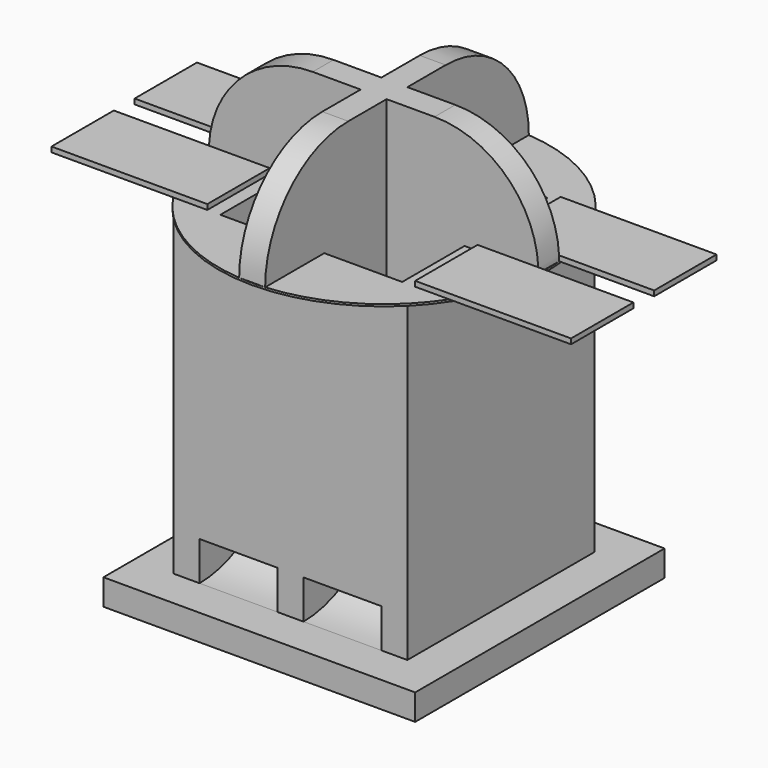
from build123d import *

# Parameters (mm, degrees)
F0_W          = 76.2
F0_H          = 76.2
F1_DEPTH      = 6.35
F2_W          = 57.15
F2_H          = 57.15
F3_DEPTH      = 76.2
F4_W          = 19.05
F4_H          = 19.05
F5_DEPTH      = 76.2
F5_DEPTH_BACK = 25.4
F7_W          = 19.05
F7_H          = 9.525
F6_W          = 19.05
F6_H          = 9.525
F8_DEPTH      = 6.35
F9_DEPTH      = 6.35
F10_R         = 25.4
F12_DEPTH     = 0.508
F13_DEPTH     = 25.4
F15_DEPTH     = 1.27
F16_W         = 6.35
F16_H         = 6.35
F17_DEPTH     = 25.4
F18_T1_DEPTH  = 6.35
F18_T3_DEPTH  = 6.35


# Not quite as in the source:
# - a fillet or chamfer that OpenCascade refuses, or shapes differently, is made with other operations: its cross-section is extruded or revolved along the edge and cut away or added


with BuildPart() as f1:
    # F0 (on Top) → F1 (new body)
    with BuildSketch(Plane.XY):
        with Locations((-41.2033051252, 20.37120983)):
            Rectangle(F0_W, F0_H)
    extrude(amount=F1_DEPTH)

    # F2 (on face) → F3 (join)
    with BuildSketch(Plane.XY.offset(6.35)):
        with Locations((-41.2033051252, 20.37120983)):
            Rectangle(F2_W, F2_H)
    extrude(amount=F3_DEPTH)

    # F4 (on face) → F5 (cut, two sides)
    with BuildSketch(Plane.XY.offset(82.55)) as f5_sk:
        with Locations((-53.9033051252, 33.07120983)):
            Rectangle(F4_W, F4_H)
        with Locations((-28.5033051252, 33.07120983)):
            Rectangle(F4_W, F4_H)
        with Locations((-28.5033051252, 7.67120983)):
            Rectangle(F4_W, F4_H)
        with Locations((-53.9033051252, 7.67120983)):
            Rectangle(F4_W, F4_H)
    extrude(amount=-F5_DEPTH, mode=Mode.SUBTRACT)
    extrude(f5_sk.sketch, amount=F5_DEPTH_BACK, mode=Mode.SUBTRACT)

    # F7 (on face) + F6 (on face) → F8 (cut)
    with BuildSketch(Plane(origin=(0, 48.94620983, 0), x_dir=(-1, 0, 0), z_dir=(0, 1, 0))):
        with Locations((28.5033051252, 11.1125)):
            Rectangle(F7_W, F7_H)
        with Locations((53.9033051252, 11.1125)):
            Rectangle(F7_W, F7_H)
    with BuildSketch(Plane.XZ.offset(8.20379017)):
        with Locations((-28.5033051252, 11.1125)):
            Rectangle(F6_W, F6_H)
        with Locations((-53.9033051252, 11.1125)):
            Rectangle(F6_W, F6_H)
    extrude(amount=-F8_DEPTH, dir=(0, 1, 0), mode=Mode.SUBTRACT)

    # F6 (on face) → F9 (cut)
    with BuildSketch(Plane.XZ.offset(8.20379017)):
        with Locations((-53.9033051252, 11.1125)):
            Rectangle(F6_W, F6_H)
        with Locations((-28.5033051252, 11.1125)):
            Rectangle(F6_W, F6_H)
    extrude(amount=-F9_DEPTH, mode=Mode.SUBTRACT)

    # F10
    f10_edges = [f1.edges().sort_by_distance(p)[0] for p in [
        (-53.903305, 17.19621, 6.35),
        (-28.503305, 17.19621, 6.35),
        (-53.903305, 23.54621, 6.35),
        (-28.503305, 23.54621, 6.35),
    ]]
    fillet(f10_edges, radius=F10_R)

    # F11 (on face) → F12 (join)
    with BuildSketch(Plane.XY.offset(82.55)):
        with BuildLine():
            ThreePointArc((-41.2033051252, -20.0399427148), (-12.6283051252, -8.20379017), (-0.7921525804, 20.37120983))
            ThreePointArc((-0.7921525804, 20.37120983), (-12.6283051252, 48.94620983), (-41.2033051252, 60.7823623749))
            Line((-41.2033051252, 60.7823623749), (-41.2033051252, -20.0399427148))
        make_face()
        with BuildLine():
            Line((-41.2033051252, -20.0399427148), (-41.2033051252, 60.7823623749))
            ThreePointArc((-41.2033051252, 60.7823623749), (-81.61445767, 20.37120983), (-41.2033051252, -20.0399427148))
        make_face()
    extrude(amount=F12_DEPTH)

    # F4 (on face) → F13 (cut)
    with BuildSketch(Plane.XY.offset(82.55)):
        with Locations((-53.9033051252, 33.07120983)):
            Rectangle(F4_W, F4_H)
        with Locations((-28.5033051252, 33.07120983)):
            Rectangle(F4_W, F4_H)
        with Locations((-28.5033051252, 7.67120983)):
            Rectangle(F4_W, F4_H)
        with Locations((-53.9033051252, 7.67120983)):
            Rectangle(F4_W, F4_H)
    extrude(amount=F13_DEPTH, mode=Mode.SUBTRACT)

    # F14 (on face) → F15 (join)
    with BuildSketch(Plane.XY.offset(83.058)):
        with BuildLine():
            ThreePointArc((-81.4895388162, 23.54620983), (-79.4275512549, 33.4848766636), (-74.9540180807, 42.59620983))
            Line((-74.9540180807, 42.59620983), (-104.7033051252, 42.59620983))
            Line((-104.7033051252, 42.59620983), (-104.7033051252, 23.54620983))
            Line((-104.7033051252, 23.54620983), (-81.4895388162, 23.54620983))
        make_face()
        with BuildLine():
            Line((-104.7033051252, -1.85379017), (-74.9540180807, -1.85379017))
            ThreePointArc((-74.9540180807, -1.85379017), (-79.4275512549, 7.2575429965), (-81.4895388162, 17.19620983))
            Line((-81.4895388162, 17.19620983), (-104.7033051252, 17.19620983))
            Line((-104.7033051252, 17.19620983), (-104.7033051252, -1.85379017))
        make_face()
        with BuildLine():
            Line((-66.6033051252, 42.59620983), (-74.9540180807, 42.59620983))
            ThreePointArc((-74.9540180807, 42.59620983), (-79.4275512549, 33.4848766636), (-81.4895388162, 23.54620983))
            Line((-81.4895388162, 23.54620983), (-66.6033051252, 23.54620983))
            Line((-66.6033051252, 23.54620983), (-66.6033051252, 42.59620983))
        make_face()
        with BuildLine():
            ThreePointArc((-81.4895388162, 17.19620983), (-79.4275512549, 7.2575429965), (-74.9540180807, -1.85379017))
            Line((-74.9540180807, -1.85379017), (-66.6033051252, -1.85379017))
            Line((-66.6033051252, -1.85379017), (-66.6033051252, 17.19620983))
            Line((-66.6033051252, 17.19620983), (-81.4895388162, 17.19620983))
        make_face()
        with BuildLine():
            Line((-15.8033051252, 42.59620983), (-15.8033051252, 23.54620983))
            Line((-15.8033051252, 23.54620983), (-0.9170714343, 23.54620983))
            ThreePointArc((-0.9170714343, 23.54620983), (-2.9790589956, 33.4848766636), (-7.4525921698, 42.59620983))
            Line((-7.4525921698, 42.59620983), (-15.8033051252, 42.59620983))
        make_face()
        with BuildLine():
            ThreePointArc((-7.4525921698, -1.85379017), (-2.9790589956, 7.2575429965), (-0.9170714343, 17.19620983))
            Line((-0.9170714343, 17.19620983), (-15.8033051252, 17.19620983))
            Line((-15.8033051252, 17.19620983), (-15.8033051252, -1.85379017))
            Line((-15.8033051252, -1.85379017), (-7.4525921698, -1.85379017))
        make_face()
        with BuildLine():
            ThreePointArc((-7.4525921698, 42.59620983), (-2.9790589956, 33.4848766636), (-0.9170714343, 23.54620983))
            Line((-0.9170714343, 23.54620983), (22.2966948748, 23.54620983))
            Line((22.2966948748, 23.54620983), (22.2966948748, 42.59620983))
            Line((22.2966948748, 42.59620983), (-7.4525921698, 42.59620983))
        make_face()
        with BuildLine():
            Line((22.2966948748, 17.19620983), (-0.9170714343, 17.19620983))
            ThreePointArc((-0.9170714343, 17.19620983), (-2.9790589956, 7.2575429965), (-7.4525921698, -1.85379017))
            Line((-7.4525921698, -1.85379017), (22.2966948748, -1.85379017))
            Line((22.2966948748, -1.85379017), (22.2966948748, 17.19620983))
        make_face()
    extrude(amount=F15_DEPTH)

    # F16 (on face) → F17 (join)
    with BuildSketch(Plane.XY.offset(83.058)):
        Polygon((-44.3783051252, 42.59620983), (-44.3783051252, 23.54620983), (-38.0283051252, 23.54620983), (-38.0283051252, 42.59620983), (-38.0283051252, 60.657443521), (-44.3783051252, 60.657443521), align=None)
        Polygon((-81.4895388162, 23.54620983), (-81.4895388162, 17.19620983), (-66.6033051252, 17.19620983), (-63.4283051252, 17.19620983), (-44.3783051252, 17.19620983), (-44.3783051252, 23.54620983), (-63.4283051252, 23.54620983), (-66.6033051252, 23.54620983), align=None)
        Polygon((-38.0283051252, 23.54620983), (-38.0283051252, 17.19620983), (-18.9783051252, 17.19620983), (-15.8033051252, 17.19620983), (-0.9170714343, 17.19620983), (-0.9170714343, 23.54620983), (-15.8033051252, 23.54620983), (-18.9783051252, 23.54620983), align=None)
        Polygon((-38.0283051252, 17.19620983), (-44.3783051252, 17.19620983), (-44.3783051252, -1.85379017), (-44.3783051252, -19.9150238609), (-38.0283051252, -19.9150238609), (-38.0283051252, -1.85379017), align=None)
        with Locations((-41.2033051252, 20.37120983)):
            Rectangle(F16_W, F16_H)
    extrude(amount=F17_DEPTH)

    # F18: fillet of radius 25.4 on 4 edges, made by hand

    # F18_s2 → F18_t1 (cut)
    with BuildSketch(Plane.YZ.offset(-44.3783051252)):
        with BuildLine():
            ThreePointArc((5.4849761391, 108.458), (-12.475536103, 101.0185122421), (-19.9150238609, 83.058))
            Line((-19.9150238609, 83.058), (-20.4230238609, 83.058))
            Line((-20.4230238609, 83.058), (-20.4230238609, 108.966))
            Line((-20.4230238609, 108.966), (5.4849761391, 108.966))
            Line((5.4849761391, 108.966), (5.4849761391, 108.458))
        make_face()
        with BuildLine():
            ThreePointArc((35.257443521, 108.458), (53.2179557631, 101.0185122421), (60.657443521, 83.058))
            Line((60.657443521, 83.058), (61.165443521, 83.058))
            Line((61.165443521, 83.058), (61.165443521, 108.966))
            Line((61.165443521, 108.966), (35.257443521, 108.966))
            Line((35.257443521, 108.966), (35.257443521, 108.458))
        make_face()
    extrude(amount=F18_T1_DEPTH, mode=Mode.SUBTRACT)

    # F18_s4 → F18_t3 (cut)
    with BuildSketch(Plane.XZ.offset(-23.54620983)):
        with BuildLine():
            ThreePointArc((-0.9170714343, 83.058), (-8.3565591922, 101.0185122421), (-26.3170714343, 108.458))
            Line((-26.3170714343, 108.458), (-26.3170714343, 108.966))
            Line((-26.3170714343, 108.966), (-0.4090714343, 108.966))
            Line((-0.4090714343, 108.966), (-0.4090714343, 83.058))
            Line((-0.4090714343, 83.058), (-0.9170714343, 83.058))
        make_face()
        with BuildLine():
            ThreePointArc((-56.0895388162, 108.458), (-74.0500510583, 101.0185122421), (-81.4895388162, 83.058))
            Line((-81.4895388162, 83.058), (-81.9975388162, 83.058))
            Line((-81.9975388162, 83.058), (-81.9975388162, 108.966))
            Line((-81.9975388162, 108.966), (-56.0895388162, 108.966))
            Line((-56.0895388162, 108.966), (-56.0895388162, 108.458))
        make_face()
    extrude(amount=F18_T3_DEPTH, mode=Mode.SUBTRACT)


solid = f1.part
